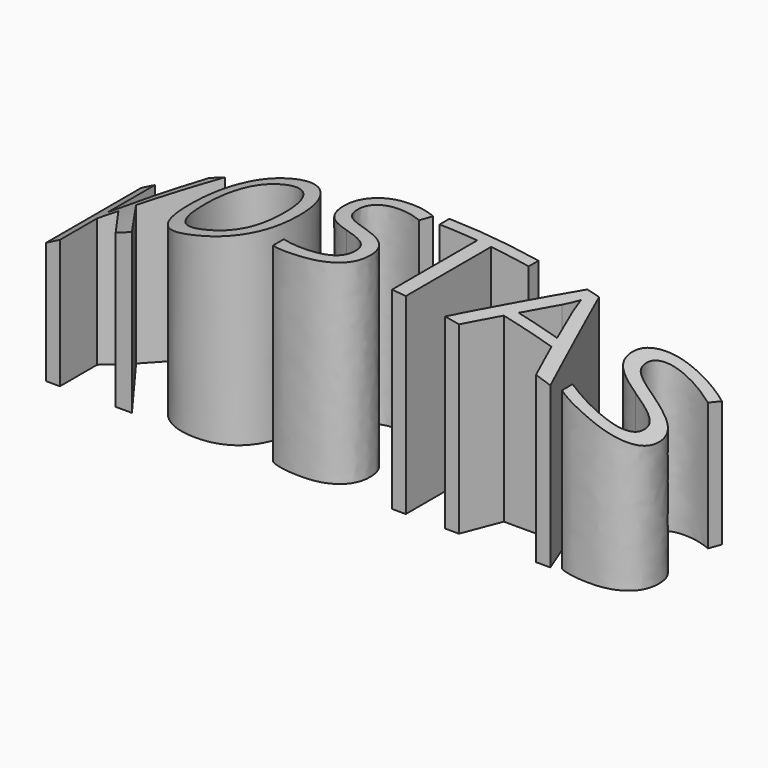
from build123d import *

# Parameters (mm, degrees)
F0_TEXT_SIZE = 10.3625300754
F1_DEPTH     = 12.7
F3_DEPTH     = 12.7


# Not quite as in the source:
# - Text() gives the source's letters only with a copy of the font that has no kerning and outlines rounded to 1/6400 em; it was checked with that copy


with BuildPart() as f1:
    # F0 (on Top) → F1 (new body)
    with BuildSketch(Plane.XY):
        with Locations((2.488389607, 0)):
            Text('KOSTAS', F0_TEXT_SIZE, font='Open Sans', text_align=(TextAlign.LEFT, TextAlign.BOTTOM))
    extrude(amount=F1_DEPTH)

    # F2 (on Front) → F3 (cut, symmetric)
    with BuildSketch(Plane.XZ):
        with BuildLine():
            ThreePointArc((-8.8307970597, -2.5191084225), (17.0119945192, 11.8311675561), (45.6046082041, 4.3316515771))
            Line((45.6046082041, 4.3316515771), (51.5748672187, 18.9622920007))
            Line((51.5748672187, 18.9622920007), (-8.8307970597, 32.5354619238))
            Line((-8.8307970597, 32.5354619238), (-8.8307970597, -2.5191084225))
        make_face()
    extrude(amount=F3_DEPTH, both=True, mode=Mode.SUBTRACT)


solid = f1.part
